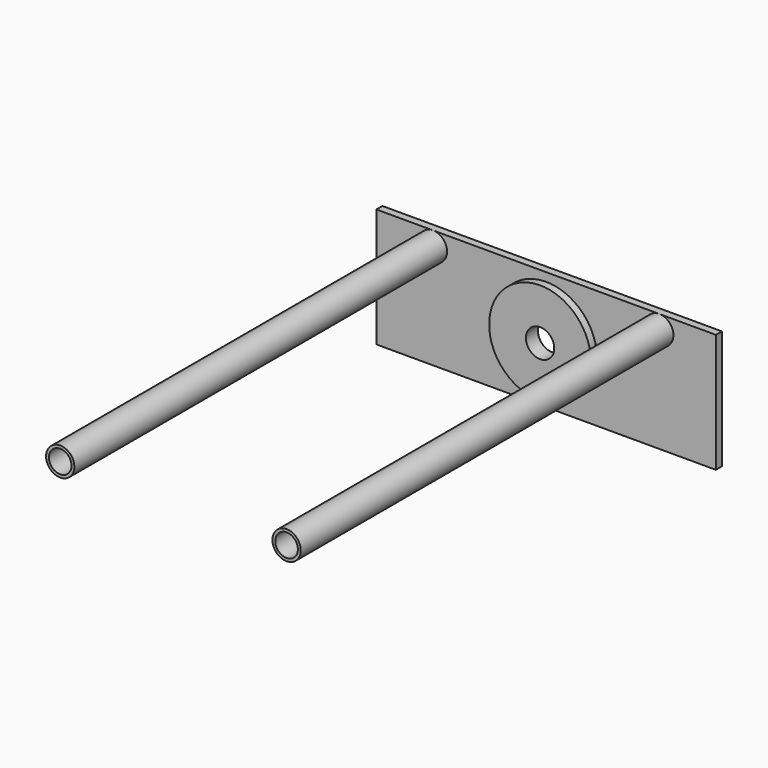
from build123d import *

# Parameters (mm, degrees)
F0_W     = 180
F0_H     = 63
F1_DEPTH = 4
F2_R     = 27
F3_DEPTH = 4
F4_DEPTH = 247
F5_R     = 7.5
F6_DEPTH = 25
F7_T     = 1.5


# Not quite as in the source:
# - a shell that OpenCascade refuses in one call is made with other operations: the cavity is built on its own and cut out


with BuildPart() as f1:
    # F0 (on Front) → F1 (new body)
    with BuildSketch(Plane.XZ):
        with Locations((90, -31.5)):
            Rectangle(F0_W, F0_H)
    extrude(amount=F1_DEPTH)

    # F2 (on face) → F3 (join)
    with BuildSketch(Plane.XZ.offset(4)):
        with Locations((90, -31.5)):
            Circle(F2_R)
    extrude(amount=F3_DEPTH)

    # F2 (on face) → F4 (join)
    with BuildSketch(Plane.XZ.offset(4)):
        with BuildLine():
            ThreePointArc((37.5, -7.5), (35.3033008593, -2.1966991415), (30.0000000011, 0))
            ThreePointArc((30.0000000011, 0), (24.6966991407, -12.8033008585), (37.5, -7.5))
        make_face()
        with BuildLine():
            ThreePointArc((150, 0), (144.6966991411, -12.8033008589), (157.5, -7.5))
            ThreePointArc((157.5, -7.5), (155.3033008589, -2.1966991411), (150, 0))
        make_face()
    extrude(amount=F4_DEPTH)

    # F5 (on face) → F6 (cut)
    with BuildSketch(Plane.XZ.offset(8)):
        with Locations((90, -31.5)):
            Circle(F5_R)
    extrude(amount=-F6_DEPTH, mode=Mode.SUBTRACT)

    # F7: shell of thickness 1.5, made by hand


with BuildPart() as f7_core1:
    # F7_t2: copy of F1
    add(f1.part)

    # the walls: a layer under each face that stays
    f7_faces = [f7_core1.faces().sort_by_distance(p)[0] for p in [
        (90, -2, 0),
        (180, -2, -31.5),
        (0, -2, -31.5),
        (30, 0, -52.5),
        (30, -4, -52.5),
        (90, -2, -63),
        (82.5, -4, -31.5),
        (63, -6, -31.5),
        (29.9999999989, -127.5, -15),
        (150, -127.5, -15),
        (72, -8, -49.5),
    ]]
    thicken(f7_faces, amount=-F7_T, mode=Mode.SUBTRACT)

    # F7_s3 → F7_t4 (revolve, cut)
    with BuildSketch(Plane.XY.offset(-31.5)):
        Polygon((117.015, -4.015), (117, -2.5), (115.5, -2.5), (115.5, -4), align=None)
    revolve(axis=Axis((90, -4, -31.5), (0, -1, 0)), mode=Mode.SUBTRACT)

    # F7_s5 → F7_t6 (revolve, cut)
    with BuildSketch(Plane.YZ.offset(30)):
        Polygon((-4.015, 0.015), (-2.5, 0), (-2.5, -1.5), (-4, -1.5), align=None)
    revolve(axis=Axis((30, -4, -7.5), (0, -1, 0)), mode=Mode.SUBTRACT)

    # F7_s7 → F7_t8 (revolve, cut)
    with BuildSketch(Plane.YZ.offset(150)):
        Polygon((-4.015, 0.015), (-2.5, 0), (-2.5, -1.5), (-4, -1.5), align=None)
    revolve(axis=Axis((150, -4, -7.5), (0, -1, 0)), mode=Mode.SUBTRACT)


with BuildPart() as f1_1:
    add(f1.part)

    # what is left inside the walls is the cavity
    f7_cavity = [f7_core1.part.solids().sort_by_distance(p)[0] for p in [
        (90, -1.515, -41.5),
    ]]
    add(f7_cavity, mode=Mode.SUBTRACT)


solid = f1_1.part
